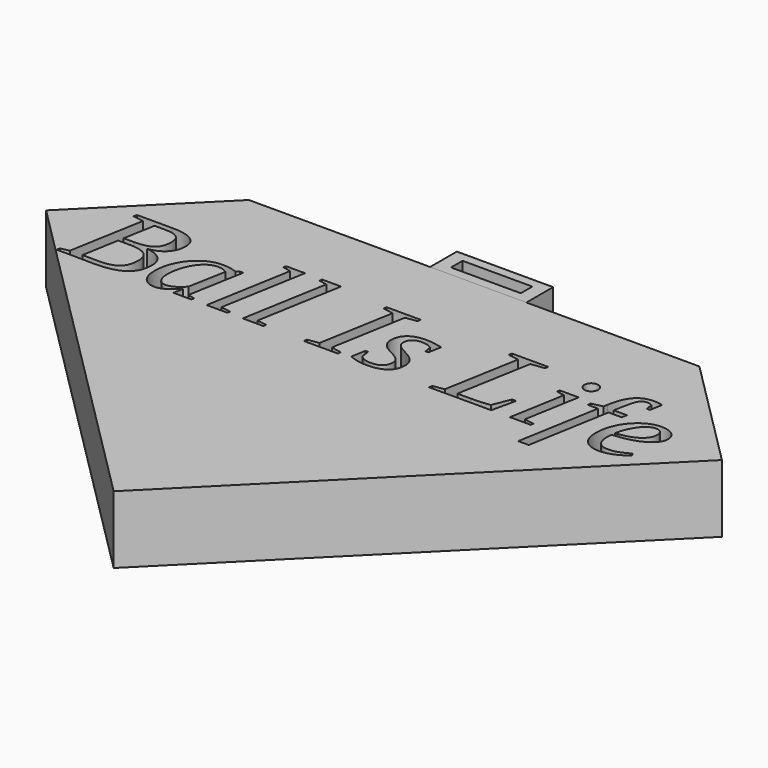
from build123d import *

# Parameters (mm, degrees)
F0_W         = 76.2
F0_H         = 50.8
F1_DEPTH     = 7.62
F2_SIZE      = 12.7
F3_SIZE      = 12.7
F4_SIZE      = 38.09999
F5_SIZE      = 38.09999
F6_TEXT_SIZE = 14.6419671541
F7_DEPTH     = 6.35
F8_W         = 10.8538353816
F8_H         = 7.5882580131
F9_DEPTH     = 3.81
F10_W        = 7.8690280207
F10_H        = 1.6280785203
F11_DEPTH    = 25.4


# Not quite as in the source:
# - a fillet or chamfer is up to 0.001 mm smaller than in the source, because OpenCascade refuses the exact size
# - Text() gives the source's letters only with a copy of the font that has no kerning and outlines rounded to 1/6400 em; it was checked with that copy


with BuildPart() as f1:
    # F0 (on Top) → F1 (new body)
    with BuildSketch(Plane.XY):
        with Locations((2.1643005311, 13.7271398962)):
            Rectangle(F0_W, F0_H)
    extrude(amount=F1_DEPTH)

    # F2
    f2_edges = [f1.edges().sort_by_distance(p)[0] for p in [
        (-35.935699, 39.12714, 3.81),
    ]]
    chamfer(f2_edges, length=F2_SIZE)

    # F3
    f3_edges = [f1.edges().sort_by_distance(p)[0] for p in [
        (40.264301, 39.12714, 3.81),
    ]]
    chamfer(f3_edges, length=F3_SIZE)

    # F4 (size 38.1 in the source; OpenCascade refuses exactly that, so slightly less here)
    f4_edges = [f1.edges().sort_by_distance(p)[0] for p in [
        (40.264301, -11.67286, 3.81),
    ]]
    chamfer(f4_edges, length=F4_SIZE)

    # F5 (size 38.1 in the source; OpenCascade refuses exactly that, so slightly less here)
    f5_edges = [f1.edges().sort_by_distance(p)[0] for p in [
        (-35.935699, -11.67286, 3.81),
    ]]
    chamfer(f5_edges, length=F5_SIZE)

    # F6 (on face) → F7 (cut)
    with BuildSketch(Plane.XY.offset(7.62)):
        with Locations((-30.6645912934, 21.1560317208)):
            Text('Ball Is Life', F6_TEXT_SIZE, font='Tinos', font_style=FontStyle.ITALIC, text_align=(TextAlign.LEFT, TextAlign.BOTTOM))
    extrude(amount=-F7_DEPTH, mode=Mode.SUBTRACT)

    # F8 (on face) → F9 (join)
    with BuildSketch(Plane(origin=(0, 39.1271398962, 0), x_dir=(-1, 0, 0), z_dir=(0, 1, 0))):
        with Locations((-2.5955669116, 3.7941290066)):
            Rectangle(F8_W, F8_H)
    extrude(amount=F9_DEPTH)

    # F10 (on face) → F11 (cut)
    with BuildSketch(Plane.XY.offset(7.5882580131)):
        with Locations((2.5955669116, 41.0624630749)):
            Rectangle(F10_W, F10_H)
    extrude(amount=-F11_DEPTH, mode=Mode.SUBTRACT)


solid = f1.part
